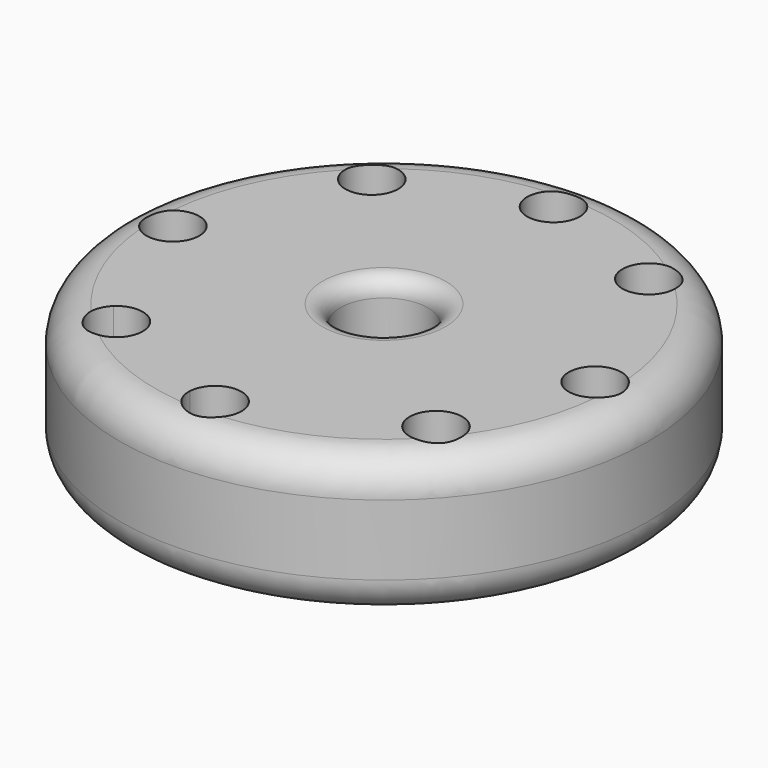
from build123d import *

# Parameters (mm, degrees)
F0_R     = 38.1
F0_R_2   = 3.81
F0_R_3   = 6.35
F1_DEPTH = 20.32
F3_R     = 2.54


# Not quite as in the source:
# - a fillet or chamfer that OpenCascade refuses, or shapes differently, is made with other operations: its cross-section is extruded or revolved along the edge and cut away or added


with BuildPart() as f1:
    # F0 (on Top) → F1 (new body)
    with BuildSketch(Plane.XY):
        Circle(F0_R)
        with BuildLine():
            ThreePointArc((-23.4644098568, -19.406517819), (-19.3435161595, -18.6884333945), (-17.0472681142, -22.1848108083))
            ThreePointArc((-17.0472681142, -22.1848108083), (-17.2730365429, -23.4768572636), (-17.923585197, -24.6157786282))
            ThreePointArc((-17.923585197, -24.6157786282), (-23.4670107891, -24.960660799), (-23.4644098568, -19.406517819))
        make_face(mode=Mode.SUBTRACT)
        with BuildLine():
            ThreePointArc((3.8025365247, -30.2114577564), (3.8081336741, -30.3305798595), (3.81, -30.4498187809))
            ThreePointArc((3.81, -30.4498187809), (-0.1192389213, -34.2579524549), (-3.8025365247, -30.2114577564))
            ThreePointArc((-3.8025365247, -30.2114577564), (0, -26.6398187809), (3.8025365247, -30.2114577564))
        make_face(mode=Mode.SUBTRACT)
        with Locations((23.2410902589, -19.6734132108)):
            Circle(F0_R_2, mode=Mode.SUBTRACT)
        with Locations((-30.4498187809, 0)):
            Circle(F0_R_2, mode=Mode.SUBTRACT)
        with Locations((-20.0773663918, 22.8930299995)):
            Circle(F0_R_2, mode=Mode.SUBTRACT)
        Circle(F0_R_3, mode=Mode.SUBTRACT)
        with Locations((30.4498187809, 0)):
            Circle(F0_R_2, mode=Mode.SUBTRACT)
        with Locations((0.0908500673, 30.4496832504)):
            Circle(F0_R_2, mode=Mode.SUBTRACT)
        with Locations((19.4666116643, 23.4145786658)):
            Circle(F0_R_2, mode=Mode.SUBTRACT)
    extrude(amount=F1_DEPTH)

    # F2: fillet of radius 5.08 on 2 edges, made by hand

    # F2_s1 → F2_t2 (revolve, cut)
    with BuildSketch(Plane.XZ):
        with BuildLine():
            ThreePointArc((38.1, 15.24), (36.6121024484, 18.8321024484), (33.02, 20.32))
            Line((33.02, 20.32), (38.1, 20.32))
            Line((38.1, 20.32), (38.1, 15.24))
        make_face()
    revolve(axis=Axis((0, 0, 20.32), (0, 0, 1)), mode=Mode.SUBTRACT)

    # F2_s3 → F2_t4 (revolve, cut)
    with BuildSketch(Plane.XZ):
        with BuildLine():
            ThreePointArc((38.1, 5.08), (36.6121024484, 1.4878975516), (33.02, 0))
            Line((33.02, 0), (38.1, 0))
            Line((38.1, 0), (38.1, 5.08))
        make_face()
    revolve(axis=Axis((0, 0, 0), (0, 0, 1)), mode=Mode.SUBTRACT)

    # F3
    f3_edges = [f1.edges().sort_by_distance(p)[0] for p in [
        (6.35, 0, 10.16),
        (-6.35, 0, 0),
        (-6.35, 0, 20.32),
    ]]
    fillet(f3_edges, radius=F3_R)


solid = f1.part
